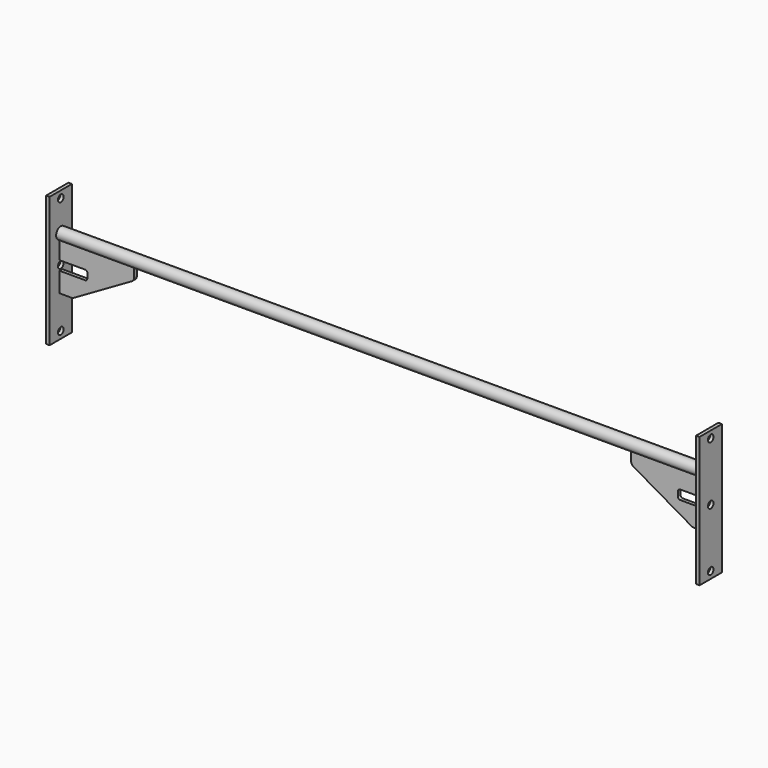
from build123d import *

# Parameters (mm, degrees)
F0_W          = 9.525
F0_H          = 355.6
F1_DEPTH      = 38.1
F1_DEPTH_BACK = 38.1
F2_R          = 15.875
F3_DEPTH      = 879.475
F3_DEPTH_BACK = 879.475
F4_R          = 9.525
F5_DEPTH      = 1778.001
F7_DEPTH      = 4.7625
F7_DEPTH_BACK = 4.7625


# Not quite as in the source:
# - a length typed as a fraction of an inch, garbled in the dataset ("3 / 203.2 mm" for 3/8 in), is restored


with BuildPart() as f1:
    # F0 (on Front) → F1 (new body, two sides)
    with BuildSketch(Plane.XZ) as f1_sk:
        with Locations((-884.2375, 0)):
            Rectangle(F0_W, F0_H)
    extrude(amount=F1_DEPTH)
    extrude(f1_sk.sketch, amount=-F1_DEPTH_BACK)


with BuildPart() as f1b:
    # F0 (on Front) → F1, piece 2 (new body, two sides)
    with BuildSketch(Plane.XZ) as f1_2_sk:
        with Locations((884.2375, 0)):
            Rectangle(F0_W, F0_H)
    extrude(amount=F1_DEPTH)
    extrude(f1_2_sk.sketch, amount=-F1_DEPTH_BACK)


with BuildPart() as f3:
    # F2 (on Right) → F3 (new body, two sides)
    with BuildSketch(Plane.YZ) as f3_sk:
        with Locations((0, 76.2)):
            Circle(F2_R)
    extrude(amount=F3_DEPTH)
    extrude(f3_sk.sketch, amount=-F3_DEPTH_BACK)


with BuildPart() as f5_tool:
    # F4 (on face) → F5 (new body, through all)
    with BuildSketch(Plane.YZ.offset(889)):
        with Locations((0, -158.75)):
            Circle(F4_R)
        Circle(F4_R)
        with Locations((0, 158.75)):
            Circle(F4_R)
    extrude(amount=-F5_DEPTH)


with BuildPart() as f1_1:
    add(f1.part)

    # F5: cut by f5_tool
    add(f5_tool.part, mode=Mode.SUBTRACT)


with BuildPart() as f1b_1:
    add(f1b.part)

    # F5: cut by f5_tool
    add(f5_tool.part, mode=Mode.SUBTRACT)


with BuildPart() as f7:
    # F6 (on Front) → F7 (new body, two sides)
    with BuildSketch(Plane.XZ) as f7_sk:
        with BuildLine():
            Line((879.475, 12.7), (879.475, 60.325))
            Line((879.4750000002, 60.325), (676.275, 60.325))
            Line((676.275, 60.325), (676.275, 37.0027863833))
            ThreePointArc((676.275, 37.0027863833), (677.9764773719, 30.6527863833), (682.625, 26.0042637552))
            Line((682.625, 26.0042637552), (840.203148376, -64.9735226281))
            ThreePointArc((840.203148376, -64.9735226281), (843.2661465032, -66.2422579939), (846.553148376, -66.675))
            Line((846.553148376, -66.675), (879.475, -66.675))
            Line((879.475, -66.675), (879.475, -12.7))
            Line((879.475, -12.7), (809.625, -12.7))
            ThreePointArc((809.625, -12.7), (805.1348719395, -10.8401280605), (803.275, -6.35))
            Line((803.275, -6.35), (803.275, 6.35))
            ThreePointArc((803.275, 6.35), (805.1348719395, 10.8401280605), (809.625, 12.7))
            Line((809.625, 12.7), (879.475, 12.7))
        make_face()
    extrude(amount=F7_DEPTH)
    extrude(f7_sk.sketch, amount=-F7_DEPTH_BACK)


with BuildPart() as f7b:
    # F6 (on Front) → F7, piece 2 (new body, two sides)
    with BuildSketch(Plane.XZ) as f7_2_sk:
        with BuildLine():
            Line((-676.275, 37.0027863833), (-676.275, 60.325))
            Line((-676.275, 60.325), (-879.4749999994, 60.325))
            Line((-879.475, 60.325), (-879.475, 12.7))
            Line((-879.475, 12.7), (-809.625, 12.7))
            ThreePointArc((-809.625, 12.7), (-805.1348719395, 10.8401280605), (-803.275, 6.35))
            Line((-803.275, 6.35), (-803.275, -6.35))
            ThreePointArc((-803.275, -6.35), (-805.1348719395, -10.8401280605), (-809.625, -12.7))
            Line((-809.625, -12.7), (-879.475, -12.7))
            Line((-879.475, -12.7), (-879.475, -66.675))
            Line((-879.475, -66.675), (-846.553148376, -66.675))
            ThreePointArc((-846.553148376, -66.675), (-843.2661465032, -66.2422579939), (-840.203148376, -64.9735226281))
            Line((-840.203148376, -64.9735226281), (-682.625, 26.0042637552))
            ThreePointArc((-682.625, 26.0042637552), (-677.9764773719, 30.6527863833), (-676.275, 37.0027863833))
        make_face()
    extrude(amount=F7_DEPTH)
    extrude(f7_2_sk.sketch, amount=-F7_DEPTH_BACK)


solid = Compound([f3.part, f1_1.part, f1b_1.part, f7.part, f7b.part])
